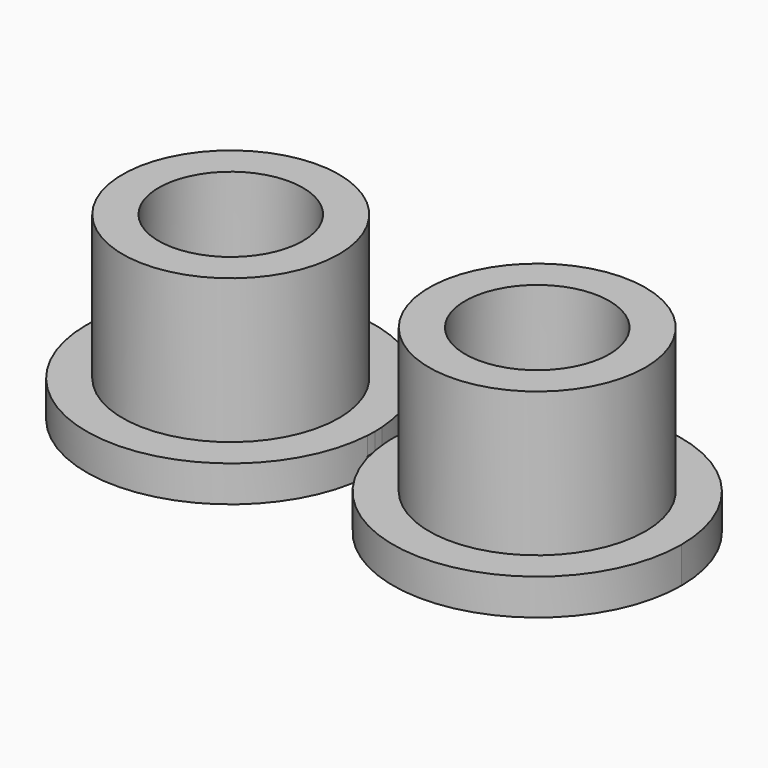
from build123d import *

# Parameters (mm, degrees)
F0_R     = 3
F0_R_2   = 2
F1_DEPTH = 5
F2_DEPTH = 1
F3_DEPTH = 0.5


# Not quite as in the source:
# - a feature names something its author has since deleted; it is built from what else it names


with BuildPart() as f1:
    # F0 (on Top) → F1 (new body)
    with BuildSketch(Plane.XY):
        with Locations((-46.8270219862, 34.2949032784)):
            Circle(F0_R)
        with Locations((-46.8270219862, 34.2949032784)):
            Circle(F0_R_2, mode=Mode.SUBTRACT)
    extrude(amount=F1_DEPTH)

    # F0 (on Top) → F2 (join)
    with BuildSketch(Plane.XY):
        with BuildLine():
            ThreePointArc((-42.8347911995, 34.0457179145), (-42.8289647614, 34.1702500531), (-42.8270219862, 34.2949032784))
            ThreePointArc((-42.8270219862, 34.2949032784), (-42.8289647614, 34.4195565036), (-42.8347911995, 34.5440886422))
            ThreePointArc((-42.8347911995, 34.5440886422), (-50.8270219862, 34.2949032784), (-42.8347911995, 34.0457179145))
        make_face()
        with Locations((-46.8270219862, 34.2949032784)):
            Circle(F0_R, mode=Mode.SUBTRACT)
        with Locations((-46.8270219862, 34.2949032784)):
            Circle(F0_R_2)
    extrude(amount=F2_DEPTH)



with BuildPart() as f1b:
    # F0 (on Top) → F1, piece 2 (new body)
    with BuildSketch(Plane.XY):
        with Locations((-38.3270219862, 34.2949032784)):
            Circle(F0_R)
        with Locations((-38.3270219862, 34.2949032784)):
            Circle(F0_R_2, mode=Mode.SUBTRACT)
    extrude(amount=F1_DEPTH)

    # F0 (on Top) → F2, piece 2 (join)
    with BuildSketch(Plane.XY):
        with BuildLine():
            ThreePointArc((-34.3270219862, 34.2949032784), (-38.202368761, 38.2929605032), (-42.319252773, 34.5440886422))
            ThreePointArc((-42.319252773, 34.5440886422), (-42.3270219862, 34.2949032784), (-42.319252773, 34.0457179145))
            ThreePointArc((-42.319252773, 34.0457179145), (-38.202368761, 30.2968460535), (-34.3270219862, 34.2949032784))
        make_face()
        with Locations((-38.3270219862, 34.2949032784)):
            Circle(F0_R, mode=Mode.SUBTRACT)
        with Locations((-38.3270219862, 34.2949032784)):
            Circle(F0_R_2)
    extrude(amount=F2_DEPTH)


with BuildPart() as f1_1:
    add(f1.part)

    add(f1b.part)  # F3 merges F1b
    # F0 (on Top) → F3 (join)
    with BuildSketch(Plane.XY):
        with BuildLine():
            ThreePointArc((-42.8347911995, 34.5440886422), (-42.8289647614, 34.4195565036), (-42.8270219862, 34.2949032784))
            ThreePointArc((-42.8270219862, 34.2949032784), (-42.8289647614, 34.1702500531), (-42.8347911995, 34.0457179145))
            Line((-42.8347911995, 34.0457179145), (-42.319252773, 34.0457179145))
            ThreePointArc((-42.319252773, 34.0457179145), (-42.3270219862, 34.2949032784), (-42.319252773, 34.5440886422))
            Line((-42.319252773, 34.5440886422), (-42.8347911995, 34.5440886422))
        make_face()
    extrude(amount=F3_DEPTH)


solid = f1_1.part
